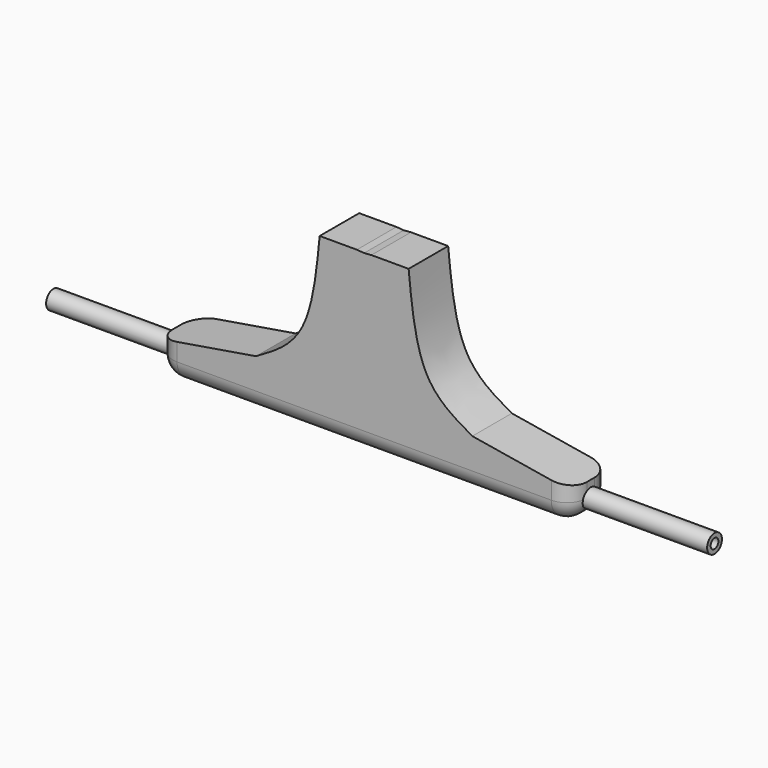
from build123d import *

# Parameters (mm, degrees)
F1_DEPTH      = 12.7
F2_R          = 2.3789042868
F3_DEPTH      = 31.75
F3_DEPTH_BACK = 138.176
F4_R          = 5.08
F5_T4_ANGLE   = 90
F5_S5_R       = 2.3789042868
F5_T6_DEPTH   = 6
F5_T10_DEPTH  = 20.32
F5_S11_R      = 2.3789042868
F5_T12_DEPTH  = 12
F5_T16_DEPTH  = 16.390593442
F5_S17_R      = 2.3789042868
F5_T18_DEPTH  = 10
F6_T1_DEPTH   = 113.968887086
F6_T6_ANGLE   = 90.0000000017
F6_S7_R       = 2.3789042868
F6_T8_DEPTH   = 6
F6_T12_DEPTH  = 16.390593442
F6_S13_R      = 2.3789042868
F6_T14_DEPTH  = 10
F7_R          = 1.2458673334
F8_DEPTH      = 25.4
F9_T4_DEPTH   = 16.390593442
F9_S5_R       = 2.3789042868
F9_T6_DEPTH   = 10
F9_T10_DEPTH  = 16.390593442
F9_S11_R      = 2.3789042868
F9_T12_DEPTH  = 10
F9_T16_ANGLE  = 90
F9_S17_R      = 2.3789042868
F9_T18_DEPTH  = 6
F9_T22_DEPTH  = 2.54
F9_S23_R      = 2.3789042868
F9_T24_DEPTH  = 5
F9_T28_ANGLE  = 90.0000000017
F9_S29_R      = 2.3789042868
F9_T30_DEPTH  = 6
F10_R         = 1.24587
F11_DEPTH     = 25.4


# Not quite as in the source:
# - a fillet or chamfer that OpenCascade refuses, or shapes differently, is made with other operations: its cross-section is extruded or revolved along the edge and cut away or added


with BuildPart() as f1:
    # F0 (on Front) → F1 (new body)
    with BuildSketch(Plane.XZ):
        with BuildLine():
            Line((-53.174443543, 7.5021637604), (0, 7.5021637604))
            Line((0, 7.5021637604), (53.174443543, 7.5021637604))
            Line((53.174443543, 7.5021637604), (53.174443543, 16.2727572024))
            Line((53.174443543, 16.2727572024), (27.8020980501, 20.4710588867))
            add(Edge.make_bspline(
                [(27.8020980501, 20.4710588867), (23.5634737704, 22.8817989501), (13.8731335003, 28.3932314282), (12.3127368707, 44.1452356637), (11.4348689094, 53.0072003603)],
                knots=[0, 0, 0, 0, 0.4374071665, 1, 1, 1, 1], degree=3))
            Line((11.4348689094, 53.0072003603), (1.8664607778, 53.0072003603))
            Line((1.8664607778, 53.0072003603), (0, 52.8586618602))
            Line((0, 52.8586618602), (-1.8664607778, 53.0072003603))
            Line((-1.8664607778, 53.0072003603), (-11.4348689094, 53.0072003603))
            add(Edge.make_bspline(
                [(-27.8020980501, 20.4710588867), (-23.5634737704, 22.8817989501), (-13.8731335003, 28.3932314282), (-12.3127368707, 44.1452356637), (-11.4348689094, 53.0072003603)],
                knots=[0, 0, 0, 0, 0.4374071665, 1, 1, 1, 1], degree=3))
            Line((-27.8020980501, 20.4710588867), (-53.174443543, 16.2727572024))
            Line((-53.174443543, 16.2727572024), (-53.174443543, 7.5021637604))
        make_face()
    extrude(amount=F1_DEPTH)

    # F2 (on face) → F3 (join, two sides)
    with BuildSketch(Plane(origin=(-53.174443543, 0, 0), x_dir=(0, -1, 0), z_dir=(-1, 0, 0))) as f3_sk:
        with Locations((6.3686654903, 12.1966870502)):
            Circle(F2_R)
    extrude(amount=F3_DEPTH)
    extrude(f3_sk.sketch, amount=-F3_DEPTH_BACK)

    # F4
    f4_edges = [f1.edges().sort_by_distance(p)[0] for p in [
        (0, 0, 7.502164),
    ]]
    fillet(f4_edges, radius=F4_R)

    # F5: fillet of radius 5.08 on 1 edges, made by hand


with BuildPart() as f5_tool2:
    # F5_s3 → F5_t4 (revolve)
    with BuildSketch(Plane.XZ.offset(5.08)):
        with BuildLine():
            ThreePointArc((-53.174443543, 12.5821637604), (-51.6865459914, 8.9900613119), (-48.094443543, 7.5021637604))
            Line((-48.094443543, 7.5021637604), (-53.174443543, 7.5021637604))
            Line((-53.174443543, 7.5021637604), (-53.174443543, 12.5821637604))
        make_face()
    revolve(axis=Axis((-53.174443543, -5.08, 12.5821637604), (1, 0, 0)), revolution_arc=F5_T4_ANGLE)

    # F5_s5 → F5_t6 (cut, symmetric)
    with BuildSketch(Plane.YZ.offset(-50.6)):
        with Locations((-6.3686654903, 12.1966870502)):
            Circle(F5_S5_R)
    extrude(amount=F5_T6_DEPTH, both=True, mode=Mode.SUBTRACT)


with BuildPart() as f1_1:
    add(f1.part)

    # F5_t1: cut F5_tool2
    add(f5_tool2.part, mode=Mode.SUBTRACT)


with BuildPart() as f5_tool8:
    # F5_s9 → F5_t10 (new body)
    with BuildSketch(Plane.XZ.offset(5.08)):
        with BuildLine():
            ThreePointArc((-48.094443543, 7.5021637604), (-51.6865459914, 8.9900613119), (-53.174443543, 12.5821637604))
            Line((-53.174443543, 12.5821637604), (-53.174443543, 7.5021637604))
            Line((-53.174443543, 7.5021637604), (-48.094443543, 7.5021637604))
        make_face()
    extrude(amount=F5_T10_DEPTH)

    # F5_s11 → F5_t12 (cut, symmetric)
    with BuildSketch(Plane.YZ.offset(-50.6)):
        with Locations((-6.3686654903, 12.1966870502)):
            Circle(F5_S11_R)
    extrude(amount=F5_T12_DEPTH, both=True, mode=Mode.SUBTRACT)


with BuildPart() as f1_2:
    add(f1_1.part)

    # F5_t7: cut F5_tool8
    add(f5_tool8.part, mode=Mode.SUBTRACT)


with BuildPart() as f5_tool14:
    # F5_s15 → F5_t16 (new body)
    with BuildSketch(Plane.XY.offset(28.9727572024)):
        with BuildLine():
            ThreePointArc((-53.174443543, -5.08), (-51.6865459914, -1.4878975516), (-48.094443543, 0))
            Line((-48.094443543, 0), (-53.174443543, 0))
            Line((-53.174443543, 0), (-53.174443543, -5.08))
        make_face()
    extrude(amount=-F5_T16_DEPTH)

    # F5_s17 → F5_t18 (cut, symmetric)
    with BuildSketch(Plane.YZ.offset(-50.6)):
        with Locations((-6.3686654903, 12.1966870502)):
            Circle(F5_S17_R)
    extrude(amount=F5_T18_DEPTH, both=True, mode=Mode.SUBTRACT)


with BuildPart() as f1_3:
    add(f1_2.part)

    # F5_t13: cut F5_tool14
    add(f5_tool14.part, mode=Mode.SUBTRACT)

    # F6: fillet of radius 5.08 on 1 edges, made by hand

    # F6_s2 → F6_t1 (cut)
    with BuildSketch(Plane.YZ.offset(-48.094443543)):
        with BuildLine():
            ThreePointArc((-7.62, 7.5021637604), (-11.2121024484, 8.9900613119), (-12.7, 12.5821637604))
            Line((-12.7, 12.5821637604), (-12.7, 7.5021637604))
            Line((-12.7, 7.5021637604), (-7.62, 7.5021637604))
        make_face()
    extrude(amount=F6_T1_DEPTH, mode=Mode.SUBTRACT)


with BuildPart() as f6_tool4:
    # F6_s5 → F6_t6 (revolve)
    with BuildSketch(Plane.YZ.offset(-48.0944435431)):
        with BuildLine():
            ThreePointArc((-12.7, 12.5821637604), (-11.2121024484, 8.990061312), (-7.62, 7.5021637604))
            Line((-7.62, 7.5021637604), (-12.7, 7.5021637604))
            Line((-12.7, 7.5021637604), (-12.7, 12.5821637604))
        make_face()
    revolve(axis=Axis((-48.0944435431, -12.7, 12.5821637603), (0, 1, 0)), revolution_arc=F6_T6_ANGLE)

    # F6_s7 → F6_t8 (cut, symmetric)
    with BuildSketch(Plane.YZ.offset(-50.6)):
        with Locations((-6.3686654903, 12.1966870502)):
            Circle(F6_S7_R)
    extrude(amount=F6_T8_DEPTH, both=True, mode=Mode.SUBTRACT)


with BuildPart() as f1_4:
    add(f1_3.part)

    # F6_t3: cut F6_tool4
    add(f6_tool4.part, mode=Mode.SUBTRACT)


with BuildPart() as f6_tool10:
    # F6_s11 → F6_t12 (new body)
    with BuildSketch(Plane.XY.offset(28.9727572024)):
        with BuildLine():
            ThreePointArc((-48.094443543, -12.7), (-51.6865459914, -11.2121024484), (-53.174443543, -7.62))
            Line((-53.174443543, -7.62), (-53.174443543, -12.7))
            Line((-53.174443543, -12.7), (-48.094443543, -12.7))
        make_face()
    extrude(amount=-F6_T12_DEPTH)

    # F6_s13 → F6_t14 (cut, symmetric)
    with BuildSketch(Plane.YZ.offset(-50.6)):
        with Locations((-6.3686654903, 12.1966870502)):
            Circle(F6_S13_R)
    extrude(amount=F6_T14_DEPTH, both=True, mode=Mode.SUBTRACT)


with BuildPart() as f1_5:
    add(f1_4.part)

    # F6_t9: cut F6_tool10
    add(f6_tool10.part, mode=Mode.SUBTRACT)

    # F7 (on face) → F8 (cut)
    with BuildSketch(Plane(origin=(-84.924443543, 0, 0), x_dir=(0, -1, 0), z_dir=(-1, 0, 0))):
        with Locations((6.3686654903, 12.1966870502)):
            Circle(F7_R)
    extrude(amount=-F8_DEPTH, mode=Mode.SUBTRACT)

    # F9: fillet of radius 5.08 on 2 edges, made by hand


with BuildPart() as f9_tool2:
    # F9_s3 → F9_t4 (new body)
    with BuildSketch(Plane.XY.offset(12.5821637604)):
        with BuildLine():
            ThreePointArc((53.174443543, -7.62), (51.6865459914, -11.2121024484), (48.094443543, -12.7))
            Line((48.094443543, -12.7), (53.174443543, -12.7))
            Line((53.174443543, -12.7), (53.174443543, -7.62))
        make_face()
    extrude(amount=F9_T4_DEPTH)

    # F9_s5 → F9_t6 (cut, symmetric)
    with BuildSketch(Plane.YZ.offset(50.6)):
        with Locations((-6.3686654903, 12.1966870502)):
            Circle(F9_S5_R)
    extrude(amount=F9_T6_DEPTH, both=True, mode=Mode.SUBTRACT)


with BuildPart() as f1_6:
    add(f1_5.part)

    # F9_t1: cut F9_tool2
    add(f9_tool2.part, mode=Mode.SUBTRACT)


with BuildPart() as f9_tool8:
    # F9_s9 → F9_t10 (new body)
    with BuildSketch(Plane.XY.offset(12.5821637604)):
        with BuildLine():
            ThreePointArc((53.174443543, -5.08), (51.6865459914, -1.4878975516), (48.094443543, 0))
            Line((48.094443543, 0), (53.174443543, 0))
            Line((53.174443543, 0), (53.174443543, -5.08))
        make_face()
    extrude(amount=F9_T10_DEPTH)

    # F9_s11 → F9_t12 (cut, symmetric)
    with BuildSketch(Plane.YZ.offset(50.6)):
        with Locations((-6.3686654903, 12.1966870502)):
            Circle(F9_S11_R)
    extrude(amount=F9_T12_DEPTH, both=True, mode=Mode.SUBTRACT)


with BuildPart() as f1_7:
    add(f1_6.part)

    # F9_t7: cut F9_tool8
    add(f9_tool8.part, mode=Mode.SUBTRACT)


with BuildPart() as f9_tool14:
    # F9_s15 → F9_t16 (revolve)
    with BuildSketch(Plane.XZ.offset(5.08)):
        with BuildLine():
            ThreePointArc((48.094443543, 7.5021637604), (51.6865459914, 8.9900613119), (53.174443543, 12.5821637604))
            Line((53.174443543, 12.5821637604), (53.174443543, 7.5021637604))
            Line((53.174443543, 7.5021637604), (48.094443543, 7.5021637604))
        make_face()
    revolve(axis=Axis((53.174443543, -5.08, 12.5821637604), (1, 0, 0)), revolution_arc=F9_T16_ANGLE)

    # F9_s17 → F9_t18 (cut, symmetric)
    with BuildSketch(Plane.YZ.offset(50.6)):
        with Locations((-6.3686654903, 12.1966870502)):
            Circle(F9_S17_R)
    extrude(amount=F9_T18_DEPTH, both=True, mode=Mode.SUBTRACT)


with BuildPart() as f1_8:
    add(f1_7.part)

    # F9_t13: cut F9_tool14
    add(f9_tool14.part, mode=Mode.SUBTRACT)


with BuildPart() as f9_tool20:
    # F9_s21 → F9_t22 (new body)
    with BuildSketch(Plane.XZ.offset(5.08)):
        with BuildLine():
            ThreePointArc((48.094443543, 7.5021637604), (51.6865459914, 8.9900613119), (53.174443543, 12.5821637604))
            Line((53.174443543, 12.5821637604), (53.174443543, 7.5021637604))
            Line((53.174443543, 7.5021637604), (48.094443543, 7.5021637604))
        make_face()
    extrude(amount=F9_T22_DEPTH)

    # F9_s23 → F9_t24 (cut, symmetric)
    with BuildSketch(Plane.YZ.offset(50.6)):
        with Locations((-6.3686654903, 12.1966870502)):
            Circle(F9_S23_R)
    extrude(amount=F9_T24_DEPTH, both=True, mode=Mode.SUBTRACT)


with BuildPart() as f1_9:
    add(f1_8.part)

    # F9_t19: cut F9_tool20
    add(f9_tool20.part, mode=Mode.SUBTRACT)


with BuildPart() as f9_tool26:
    # F9_s27 → F9_t28 (revolve)
    with BuildSketch(Plane.XZ.offset(7.6200000001)):
        with BuildLine():
            ThreePointArc((53.174443543, 12.5821637604), (51.6865459914, 8.990061312), (48.094443543, 7.5021637604))
            Line((48.094443543, 7.5021637604), (53.174443543, 7.5021637604))
            Line((53.174443543, 7.5021637604), (53.174443543, 12.5821637604))
        make_face()
    revolve(axis=Axis((53.174443543, -7.6200000001, 12.5821637603), (-1, 0, 0)), revolution_arc=F9_T28_ANGLE)

    # F9_s29 → F9_t30 (cut, symmetric)
    with BuildSketch(Plane.YZ.offset(50.6)):
        with Locations((-6.3686654903, 12.1966870502)):
            Circle(F9_S29_R)
    extrude(amount=F9_T30_DEPTH, both=True, mode=Mode.SUBTRACT)


with BuildPart() as f1_10:
    add(f1_9.part)

    # F9_t25: cut F9_tool26
    add(f9_tool26.part, mode=Mode.SUBTRACT)

    # F10 (on face) → F11 (cut)
    with BuildSketch(Plane.YZ.offset(85.001556457)):
        with Locations((-6.3686654903, 12.1966870502)):
            Circle(F10_R)
    extrude(amount=-F11_DEPTH, mode=Mode.SUBTRACT)


solid = f1_10.part
